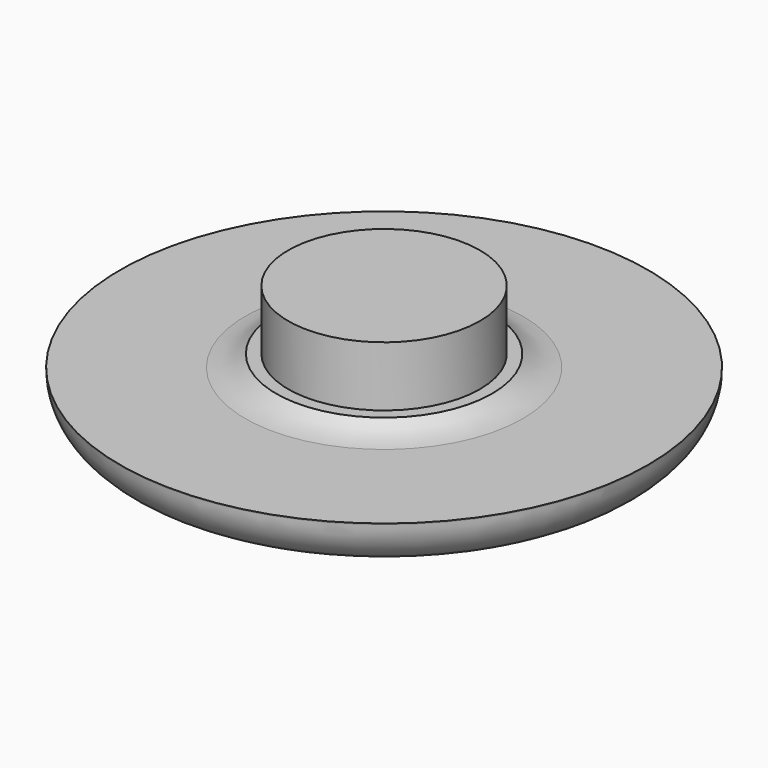
from build123d import *

# Parameters (mm, degrees)
F0_R         = 11
F1_DEPTH     = 2
F2_R         = 4.5
F3_DEPTH     = 0.5
F4_R         = 3.995
F5_DEPTH     = 2.5
F7_TEXT_SIZE = 5.2459016393
F8_DEPTH     = 1


# Not quite as in the source:
# - a fillet or chamfer that OpenCascade refuses, or shapes differently, is made with other operations: its cross-section is extruded or revolved along the edge and cut away or added
# - Text() gives the source's letters only with a copy of the font that has no kerning and outlines rounded to 1/6400 em; it was checked with that copy


with BuildPart() as f1:
    # F0 (on Top) → F1 (new body)
    with BuildSketch(Plane.XY):
        with Locations((-124.7583553195, 13.61318212)):
            Circle(F0_R)
    extrude(amount=F1_DEPTH)

    # F2 (on face) → F3 (join)
    with BuildSketch(Plane.XY.offset(2)):
        with Locations((-124.7583553195, 13.61318212)):
            Circle(F2_R)
    extrude(amount=F3_DEPTH)

    # F4 (on face) → F5 (join)
    with BuildSketch(Plane.XY.offset(2.5)):
        with Locations((-124.7583553195, 13.61318212)):
            Circle(F4_R)
    extrude(amount=F5_DEPTH)

    # F6: fillet of radius 2 on 2 edges, made by hand

    # F6_s1 → F6_t2 (revolve)
    with BuildSketch(Plane.XZ.offset(-13.61318212)):
        with BuildLine():
            ThreePointArc((-118.9351147195, 1.9996), (-119.642533578, 2.1287949759), (-120.2586198399, 2.4996999517))
            Line((-120.2586198399, 2.4996999517), (-120.3909703519, 2.3495733784))
            ThreePointArc((-120.3909703519, 2.3495733784), (-120.458491888, 2.2498499759), (-120.458491888, 2))
            Line((-120.458491888, 2), (-120.2583553195, 1.7998634315))
            ThreePointArc((-120.2583553195, 1.7998634315), (-119.5967350195, 1.7998634315), (-118.9351147195, 1.7994634315))
            Line((-118.9351147195, 1.7994634315), (-118.9351147195, 1.9996))
        make_face()
    revolve(axis=Axis((-124.7583553195, 13.61318212, 2), (0, 0, 1)))

    # F6_s3 → F6_t4 (revolve, cut)
    with BuildSketch(Plane.XZ.offset(-13.61318212)):
        with BuildLine():
            ThreePointArc((-113.7579553195, 1.999999807), (-114.3444830549, 0.5854449892), (-115.7593207719, -0.0004))
            Line((-115.7593207719, -0.0004), (-115.7593207719, -0.2005365685))
            ThreePointArc((-115.7593207719, -0.2005365685), (-114.7588380457, -0.2001365685), (-113.7583553195, -0.2001365685))
            Line((-113.7583553195, -0.2001365685), (-113.558218751, 0))
            ThreePointArc((-113.558218751, 0), (-113.558218751, 0.9999999035), (-113.5578187743, 1.9999032191))
            Line((-113.5578187743, 1.9999032191), (-113.7579553195, 1.999999807))
        make_face()
    revolve(axis=Axis((-124.7583553195, 13.61318212, 0), (0, 0, 1)), mode=Mode.SUBTRACT)

    # F7 (on face) → F8 (cut)
    with BuildSketch(Plane(origin=(0, 0, 0), x_dir=(1, 0, 0), z_dir=(0, 0, -1))):
        with Locations((-132.8461730087, -15.1907329428)):
            Text('upper', F7_TEXT_SIZE, font='Open Sans', font_style=FontStyle.BOLD, text_align=(TextAlign.LEFT, TextAlign.BOTTOM))
    extrude(amount=-F8_DEPTH, mode=Mode.SUBTRACT)


solid = f1.part
